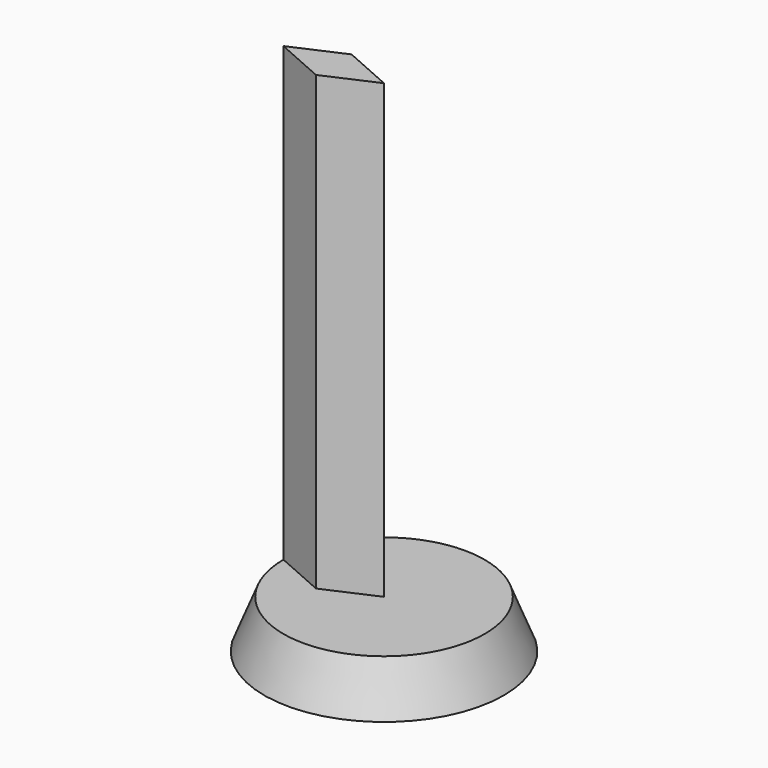
from build123d import *

# Parameters (mm, degrees)
F0_R     = 15.875
F1_DEPTH = 6.35
F2_SIZE2 = 6.34999
F2_SIZE  = 2.53999
F4_DEPTH = 59.95412


# Not quite as in the source:
# - a fillet or chamfer is up to 0.001 mm smaller than in the source, because OpenCascade refuses the exact size


with BuildPart() as f1:
    # F0 (on Top) → F1 (new body)
    with BuildSketch(Plane.XY):
        Circle(F0_R)
    extrude(amount=F1_DEPTH)

    # F2 (size 2.54 and 6.35 in the source; OpenCascade refuses exactly that, so slightly less here)
    f2_edges = [f1.edges().sort_by_distance(p)[0] for p in [
        (-15.875, 0, 6.35),
    ]]
    f2_side = f1.faces().sort_by_distance((0, 0, 6.35))[0]
    chamfer(f2_edges, length=F2_SIZE, length2=F2_SIZE2, reference=f2_side)

    # F3 (on face) → F4 (join)
    with BuildSketch(Plane.XY.offset(6.35)):
        Polygon((-6.6675, 2.9491111636), (-13.335, 0), (-6.6675, -2.9491111636), (0, 0), align=None)
    extrude(amount=F4_DEPTH)


solid = f1.part
